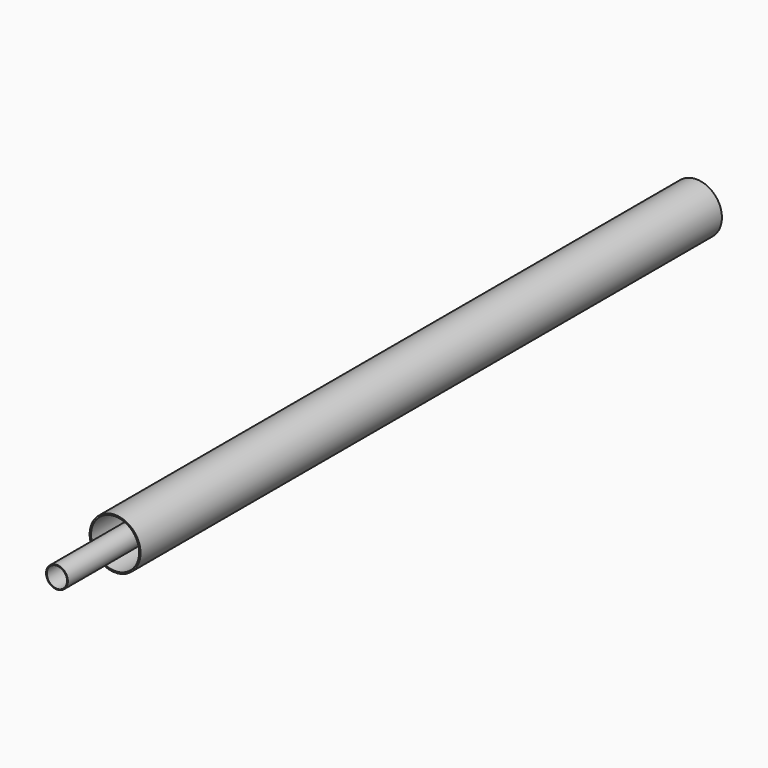
from build123d import *

# Parameters (mm, degrees)
F0_R     = 88.9
F0_R_2   = 84.1250430216
F1_DEPTH = 2540
F0_R_3   = 38.1
F0_R_4   = 35.306
F3_DEPTH = 254


# Not quite as in the source:
# - the program builds the solid bodies; features that only make, move or delete a surface that nothing else refers to are left out


with BuildPart() as f1:
    # F0 (on Front) → F1 (new body)
    with BuildSketch(Plane.XZ):
        Circle(F0_R)
        Circle(F0_R_2, mode=Mode.SUBTRACT)
    extrude(amount=F1_DEPTH)


with BuildPart() as f1b:
    # F0 (on Front) → F1, piece 2 (new body)
    with BuildSketch(Plane.XZ):
        Circle(F0_R_3)
        Circle(F0_R_4, mode=Mode.SUBTRACT)
    extrude(amount=F1_DEPTH)

    # F3 (add): a face of the model
    f3_faces = [f1b.faces().sort_by_distance(p)[0] for p in [
        (-37.0223692655, -2540, 0),
    ]]
    extrude(f3_faces, amount=F3_DEPTH)


solid = Compound([f1.part, f1b.part])
